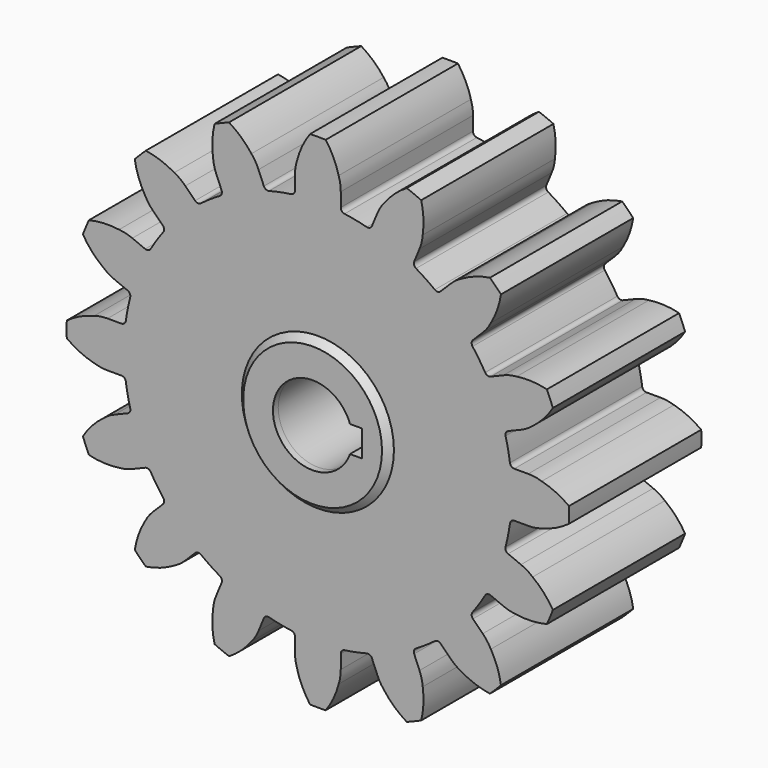
from build123d import *

# Parameters (mm, degrees)
F1_DEPTH = 25
F2_R     = 23
F3_DEPTH = 2
F4_SIZE  = 1.99999


# Not quite as in the source:
# - a fillet or chamfer is up to 0.001 mm smaller than in the source, because OpenCascade refuses the exact size
# - a pattern or mirror of a feature is missing from the dataset's text; its kind, count and spacing are read off the source's solid


with BuildPart() as f1:
    # F0 (on Front) → F1 (new body, symmetric)
    with BuildSketch(Plane.XZ):
        with BuildLine():
            ThreePointArc((-43.4371387857, 52.3183999575), (-47.5930049545, 54.262886018), (-52.0415397972, 55.3866241573))
            ThreePointArc((-52.0415397972, 55.3866241573), (-53.7401153702, 53.7401153702), (-55.3866241573, 52.0415397972))
            ThreePointArc((-55.3866241573, 52.0415397972), (-54.262886018, 47.5930049545), (-52.3183999575, 43.4371387857))
            ThreePointArc((-52.3183999575, 43.4371387857), (-51.237231337, 41.6673521086), (-49.8812173358, 40.0981814687))
            Line((-49.8812173358, 40.0981814687), (-46.908040594, 37.1250047269))
            ThreePointArc((-46.908040594, 37.1250047269), (-46.5216537829, 36.2761972334), (-46.7876742236, 35.3823280854))
            ThreePointArc((-46.7876742236, 35.3823280854), (-48.7740074577, 32.5897498689), (-50.593876495, 29.6859438322))
            ThreePointArc((-50.593876495, 29.6859438322), (-51.3179022902, 29.0981040781), (-52.2499619915, 29.1302543795))
            Line((-52.2499619915, 29.1302543795), (-56.1346046105, 30.7393260373))
            ThreePointArc((-56.1346046105, 30.7393260373), (-58.10325334, 31.3916240124), (-60.1520683466, 31.7132255318))
            ThreePointArc((-60.1520683466, 31.7132255318), (-64.7357106396, 31.9193152744), (-69.2756568986, 31.2551333587))
            ThreePointArc((-69.2756568986, 31.2551333587), (-70.2148444709, 29.0839408597), (-71.086003509, 26.8845700193))
            ThreePointArc((-71.086003509, 26.8845700193), (-68.3454242596, 23.2046956968), (-64.9585722571, 20.1092986034))
            ThreePointArc((-64.9585722571, 20.1092986034), (-63.2824346573, 18.8879742341), (-61.4291454693, 17.9571736892))
            Line((-61.4291454693, 17.9571736892), (-57.5445028504, 16.3481020315))
            ThreePointArc((-57.5445028504, 16.3481020315), (-56.862703419, 15.7117699924), (-56.7664053458, 14.7841409664))
            ThreePointArc((-56.7664053458, 14.7841409664), (-57.5328645485, 11.4439982895), (-58.1029658428, 8.0647975961))
            ThreePointArc((-58.1029658428, 8.0647975961), (-58.5469219213, 7.2446318025), (-59.4203361901, 6.9176510022))
            Line((-59.4203361901, 6.9176510022), (-63.6250430618, 6.9176510022))
            ThreePointArc((-63.6250430618, 6.9176510022), (-65.6934609577, 6.7669264976), (-67.7093907815, 6.28))
            ThreePointArc((-67.7093907815, 6.28), (-72.0229912104, 4.7163181297), (-75.9631832226, 2.3653318347))
            ThreePointArc((-75.9631832226, 2.3653318347), (-76, 0), (-75.9631832226, -2.3653318347))
            ThreePointArc((-75.9631832226, -2.3653318347), (-72.0229912104, -4.7163181297), (-67.7093907815, -6.28))
            ThreePointArc((-67.7093907815, -6.28), (-65.6934609577, -6.7669264976), (-63.6250430618, -6.9176510022))
            Line((-63.6250430618, -6.9176510022), (-59.4203361901, -6.9176510022))
            ThreePointArc((-59.4203361901, -6.9176510022), (-58.5469219213, -7.2446318025), (-58.1029658428, -8.0647975961))
            ThreePointArc((-58.1029658428, -8.0647975961), (-57.5328645485, -11.4439982895), (-56.7664053458, -14.7841409664))
            ThreePointArc((-56.7664053458, -14.7841409664), (-56.862703419, -15.7117699924), (-57.5445028504, -16.3481020315))
            Line((-57.5445028504, -16.3481020315), (-61.4291454693, -17.9571736892))
            ThreePointArc((-61.4291454693, -17.9571736892), (-63.2824346573, -18.8879742341), (-64.9585722571, -20.1092986034))
            ThreePointArc((-64.9585722571, -20.1092986034), (-68.3454242596, -23.2046956968), (-71.086003509, -26.8845700193))
            ThreePointArc((-71.086003509, -26.8845700193), (-70.2148444709, -29.0839408597), (-69.2756568986, -31.2551333587))
            ThreePointArc((-69.2756568986, -31.2551333587), (-64.7357106396, -31.9193152744), (-60.1520683466, -31.7132255318))
            ThreePointArc((-60.1520683466, -31.7132255318), (-58.10325334, -31.3916240124), (-56.1346046105, -30.7393260373))
            Line((-56.1346046105, -30.7393260373), (-52.2499619915, -29.1302543795))
            ThreePointArc((-52.2499619915, -29.1302543795), (-51.3179022902, -29.0981040781), (-50.593876495, -29.6859438322))
            ThreePointArc((-50.593876495, -29.6859438322), (-48.7740074577, -32.5897498689), (-46.7876742236, -35.3823280854))
            ThreePointArc((-46.7876742236, -35.3823280854), (-46.5216537829, -36.2761972334), (-46.908040594, -37.1250047269))
            Line((-46.908040594, -37.1250047269), (-49.8812173358, -40.0981814687))
            ThreePointArc((-49.8812173358, -40.0981814687), (-51.237231337, -41.6673521086), (-52.3183999575, -43.4371387857))
            ThreePointArc((-52.3183999575, -43.4371387857), (-54.262886018, -47.5930049545), (-55.3866241573, -52.0415397972))
            ThreePointArc((-55.3866241573, -52.0415397972), (-53.7401153702, -53.7401153702), (-52.0415397972, -55.3866241573))
            ThreePointArc((-52.0415397972, -55.3866241573), (-47.5930049545, -54.262886018), (-43.4371387857, -52.3183999575))
            ThreePointArc((-43.4371387857, -52.3183999575), (-41.6673521086, -51.237231337), (-40.0981814687, -49.8812173358))
            Line((-40.0981814687, -49.8812173358), (-37.1250047269, -46.908040594))
            ThreePointArc((-37.1250047269, -46.908040594), (-36.2761972334, -46.5216537829), (-35.3823280854, -46.7876742236))
            ThreePointArc((-35.3823280854, -46.7876742236), (-32.5897498689, -48.7740074577), (-29.6859438322, -50.593876495))
            ThreePointArc((-29.6859438322, -50.593876495), (-29.0981040781, -51.3179022902), (-29.1302543795, -52.2499619915))
            Line((-29.1302543795, -52.2499619915), (-30.7393260373, -56.1346046105))
            ThreePointArc((-30.7393260373, -56.1346046105), (-31.3916240124, -58.10325334), (-31.7132255318, -60.1520683466))
            ThreePointArc((-31.7132255318, -60.1520683466), (-31.9193152744, -64.7357106396), (-31.2551333587, -69.2756568986))
            ThreePointArc((-31.2551333587, -69.2756568986), (-29.0839408597, -70.2148444709), (-26.8845700193, -71.086003509))
            ThreePointArc((-26.8845700193, -71.086003509), (-23.2046956968, -68.3454242596), (-20.1092986034, -64.9585722571))
            ThreePointArc((-20.1092986034, -64.9585722571), (-18.8879742341, -63.2824346573), (-17.9571736892, -61.4291454693))
            Line((-17.9571736892, -61.4291454693), (-16.3481020315, -57.5445028504))
            ThreePointArc((-16.3481020315, -57.5445028504), (-15.7117699924, -56.862703419), (-14.7841409664, -56.7664053458))
            ThreePointArc((-14.7841409664, -56.7664053458), (-11.4439982895, -57.5328645485), (-8.0647975961, -58.1029658428))
            ThreePointArc((-8.0647975961, -58.1029658428), (-7.2446318025, -58.5469219213), (-6.9176510022, -59.4203361901))
            Line((-6.9176510022, -59.4203361901), (-6.9176510022, -63.6250430618))
            ThreePointArc((-6.9176510022, -63.6250430618), (-6.7669264976, -65.6934609577), (-6.28, -67.7093907815))
            ThreePointArc((-6.28, -67.7093907815), (-4.7163181297, -72.0229912104), (-2.3653318347, -75.9631832226))
            ThreePointArc((-2.3653318347, -75.9631832226), (0, -76), (2.3653318347, -75.9631832226))
            ThreePointArc((2.3653318347, -75.9631832226), (4.7163181297, -72.0229912104), (6.28, -67.7093907815))
            ThreePointArc((6.28, -67.7093907815), (6.7669264976, -65.6934609577), (6.9176510022, -63.6250430618))
            Line((6.9176510022, -63.6250430618), (6.9176510022, -59.4203361901))
            ThreePointArc((6.9176510022, -59.4203361901), (7.2446318025, -58.5469219213), (8.0647975961, -58.1029658428))
            ThreePointArc((8.0647975961, -58.1029658428), (11.4439982895, -57.5328645485), (14.7841409664, -56.7664053458))
            ThreePointArc((14.7841409664, -56.7664053458), (15.7117699924, -56.862703419), (16.3481020315, -57.5445028504))
            Line((16.3481020315, -57.5445028504), (17.9571736892, -61.4291454693))
            ThreePointArc((17.9571736892, -61.4291454693), (18.8879742341, -63.2824346573), (20.1092986034, -64.9585722571))
            ThreePointArc((20.1092986034, -64.9585722571), (23.2046956968, -68.3454242596), (26.8845700193, -71.086003509))
            ThreePointArc((26.8845700193, -71.086003509), (29.0839408597, -70.2148444709), (31.2551333587, -69.2756568986))
            ThreePointArc((31.2551333587, -69.2756568986), (31.9193152744, -64.7357106396), (31.7132255318, -60.1520683466))
            ThreePointArc((31.7132255318, -60.1520683466), (31.3916240124, -58.10325334), (30.7393260373, -56.1346046105))
            Line((30.7393260373, -56.1346046105), (29.1302543795, -52.2499619915))
            ThreePointArc((29.1302543795, -52.2499619915), (29.0981040781, -51.3179022902), (29.6859438322, -50.593876495))
            ThreePointArc((29.6859438322, -50.593876495), (32.5897498689, -48.7740074577), (35.3823280854, -46.7876742236))
            ThreePointArc((35.3823280854, -46.7876742236), (36.2761972334, -46.5216537829), (37.1250047269, -46.908040594))
            Line((37.1250047269, -46.908040594), (40.0981814687, -49.8812173358))
            ThreePointArc((40.0981814687, -49.8812173358), (41.6673521086, -51.237231337), (43.4371387857, -52.3183999575))
            ThreePointArc((43.4371387857, -52.3183999575), (47.5930049545, -54.262886018), (52.0415397972, -55.3866241573))
            ThreePointArc((52.0415397972, -55.3866241573), (53.7401153702, -53.7401153702), (55.3866241573, -52.0415397972))
            ThreePointArc((55.3866241573, -52.0415397972), (54.262886018, -47.5930049545), (52.3183999575, -43.4371387857))
            ThreePointArc((52.3183999575, -43.4371387857), (51.237231337, -41.6673521086), (49.8812173358, -40.0981814687))
            Line((49.8812173358, -40.0981814687), (46.908040594, -37.1250047269))
            ThreePointArc((46.908040594, -37.1250047269), (46.5216537829, -36.2761972334), (46.7876742236, -35.3823280854))
            ThreePointArc((46.7876742236, -35.3823280854), (48.7740074577, -32.5897498689), (50.593876495, -29.6859438322))
            ThreePointArc((50.593876495, -29.6859438322), (51.3179022902, -29.0981040781), (52.2499619915, -29.1302543795))
            Line((52.2499619915, -29.1302543795), (56.1346046105, -30.7393260373))
            ThreePointArc((56.1346046105, -30.7393260373), (58.10325334, -31.3916240124), (60.1520683466, -31.7132255318))
            ThreePointArc((60.1520683466, -31.7132255318), (64.7357106396, -31.9193152744), (69.2756568986, -31.2551333587))
            ThreePointArc((69.2756568986, -31.2551333587), (70.2148444709, -29.0839408597), (71.086003509, -26.8845700193))
            ThreePointArc((71.086003509, -26.8845700193), (68.3454242596, -23.2046956968), (64.9585722571, -20.1092986034))
            ThreePointArc((64.9585722571, -20.1092986034), (63.2824346573, -18.8879742341), (61.4291454693, -17.9571736892))
            Line((61.4291454693, -17.9571736892), (57.5445028504, -16.3481020315))
            ThreePointArc((57.5445028504, -16.3481020315), (56.862703419, -15.7117699924), (56.7664053458, -14.7841409664))
            ThreePointArc((56.7664053458, -14.7841409664), (57.5328645485, -11.4439982895), (58.1029658428, -8.0647975961))
            ThreePointArc((58.1029658428, -8.0647975961), (58.5469219213, -7.2446318025), (59.4203361901, -6.9176510022))
            Line((59.4203361901, -6.9176510022), (63.6250430618, -6.9176510022))
            ThreePointArc((63.6250430618, -6.9176510022), (65.6934609577, -6.7669264976), (67.7093907815, -6.28))
            ThreePointArc((67.7093907815, -6.28), (72.0229912104, -4.7163181297), (75.9631832226, -2.3653318347))
            ThreePointArc((75.9631832226, -2.3653318347), (76, 0), (75.9631832226, 2.3653318347))
            ThreePointArc((75.9631832226, 2.3653318347), (72.0229912104, 4.7163181297), (67.7093907815, 6.28))
            ThreePointArc((67.7093907815, 6.28), (65.6934609577, 6.7669264976), (63.6250430618, 6.9176510022))
            Line((63.6250430618, 6.9176510022), (59.4203361901, 6.9176510022))
            ThreePointArc((59.4203361901, 6.9176510022), (58.5469219213, 7.2446318025), (58.1029658428, 8.0647975961))
            ThreePointArc((58.1029658428, 8.0647975961), (57.5328645485, 11.4439982895), (56.7664053458, 14.7841409664))
            ThreePointArc((56.7664053458, 14.7841409664), (56.862703419, 15.7117699924), (57.5445028504, 16.3481020315))
            Line((57.5445028504, 16.3481020315), (61.4291454693, 17.9571736892))
            ThreePointArc((61.4291454693, 17.9571736892), (63.2824346573, 18.8879742341), (64.9585722571, 20.1092986034))
            ThreePointArc((64.9585722571, 20.1092986034), (68.3454242596, 23.2046956968), (71.086003509, 26.8845700193))
            ThreePointArc((71.086003509, 26.8845700193), (70.2148444709, 29.0839408597), (69.2756568986, 31.2551333587))
            ThreePointArc((69.2756568986, 31.2551333587), (64.7357106396, 31.9193152744), (60.1520683466, 31.7132255318))
            ThreePointArc((60.1520683466, 31.7132255318), (58.10325334, 31.3916240124), (56.1346046105, 30.7393260373))
            Line((56.1346046105, 30.7393260373), (52.2499619915, 29.1302543795))
            ThreePointArc((52.2499619915, 29.1302543795), (51.3179022902, 29.0981040781), (50.593876495, 29.6859438322))
            ThreePointArc((50.593876495, 29.6859438322), (48.7740074577, 32.5897498689), (46.7876742236, 35.3823280854))
            ThreePointArc((46.7876742236, 35.3823280854), (46.5216537829, 36.2761972334), (46.908040594, 37.1250047269))
            Line((46.908040594, 37.1250047269), (49.8812173358, 40.0981814687))
            ThreePointArc((49.8812173358, 40.0981814687), (51.237231337, 41.6673521086), (52.3183999575, 43.4371387857))
            ThreePointArc((52.3183999575, 43.4371387857), (54.262886018, 47.5930049545), (55.3866241573, 52.0415397972))
            ThreePointArc((55.3866241573, 52.0415397972), (53.7401153702, 53.7401153702), (52.0415397972, 55.3866241573))
            ThreePointArc((52.0415397972, 55.3866241573), (47.5930049545, 54.262886018), (43.4371387857, 52.3183999575))
            ThreePointArc((43.4371387857, 52.3183999575), (41.6673521086, 51.237231337), (40.0981814687, 49.8812173358))
            Line((40.0981814687, 49.8812173358), (37.1250047269, 46.908040594))
            ThreePointArc((37.1250047269, 46.908040594), (36.2761972334, 46.5216537829), (35.3823280854, 46.7876742236))
            ThreePointArc((35.3823280854, 46.7876742236), (32.5897498689, 48.7740074577), (29.6859438322, 50.593876495))
            ThreePointArc((29.6859438322, 50.593876495), (29.0981040781, 51.3179022902), (29.1302543795, 52.2499619915))
            Line((29.1302543795, 52.2499619915), (30.7393260373, 56.1346046105))
            ThreePointArc((30.7393260373, 56.1346046105), (31.3916240124, 58.10325334), (31.7132255318, 60.1520683466))
            ThreePointArc((31.7132255318, 60.1520683466), (31.9193152744, 64.7357106396), (31.2551333587, 69.2756568986))
            ThreePointArc((31.2551333587, 69.2756568986), (29.0839408597, 70.2148444709), (26.8845700193, 71.086003509))
            ThreePointArc((26.8845700193, 71.086003509), (23.2046956968, 68.3454242596), (20.1092986034, 64.9585722571))
            ThreePointArc((20.1092986034, 64.9585722571), (18.8879742341, 63.2824346573), (17.9571736892, 61.4291454693))
            Line((17.9571736892, 61.4291454693), (16.3481020315, 57.5445028504))
            ThreePointArc((16.3481020315, 57.5445028504), (15.7117699924, 56.862703419), (14.7841409664, 56.7664053458))
            ThreePointArc((14.7841409664, 56.7664053458), (11.4439982895, 57.5328645485), (8.0647975961, 58.1029658428))
            ThreePointArc((8.0647975961, 58.1029658428), (7.2446318025, 58.5469219213), (6.9176510022, 59.4203361901))
            Line((6.9176510022, 59.4203361901), (6.9176510022, 63.6250430618))
            ThreePointArc((6.9176510022, 63.6250430618), (6.7669264976, 65.6934609577), (6.28, 67.7093907815))
            ThreePointArc((6.28, 67.7093907815), (4.7163181297, 72.0229912104), (2.3653318347, 75.9631832226))
            ThreePointArc((2.3653318347, 75.9631832226), (0, 76), (-2.3653318347, 75.9631832226))
            ThreePointArc((-2.3653318347, 75.9631832226), (-4.7163181297, 72.0229912104), (-6.28, 67.7093907815))
            ThreePointArc((-6.28, 67.7093907815), (-6.7669264976, 65.6934609577), (-6.9176510022, 63.6250430618))
            Line((-6.9176510022, 63.6250430618), (-6.9176510022, 59.4203361901))
            ThreePointArc((-6.9176510022, 59.4203361901), (-7.2446318025, 58.5469219213), (-8.0647975961, 58.1029658428))
            ThreePointArc((-8.0647975961, 58.1029658428), (-11.4439982895, 57.5328645485), (-14.7841409664, 56.7664053458))
            ThreePointArc((-14.7841409664, 56.7664053458), (-15.7117699924, 56.862703419), (-16.3481020315, 57.5445028504))
            Line((-16.3481020315, 57.5445028504), (-17.9571736892, 61.4291454693))
            ThreePointArc((-17.9571736892, 61.4291454693), (-18.8879742341, 63.2824346573), (-20.1092986034, 64.9585722571))
            ThreePointArc((-20.1092986034, 64.9585722571), (-23.2046956968, 68.3454242596), (-26.8845700193, 71.086003509))
            ThreePointArc((-26.8845700193, 71.086003509), (-29.0839408597, 70.2148444709), (-31.2551333587, 69.2756568986))
            ThreePointArc((-31.2551333587, 69.2756568986), (-31.9193152744, 64.7357106396), (-31.7132255318, 60.1520683466))
            ThreePointArc((-31.7132255318, 60.1520683466), (-31.3916240124, 58.10325334), (-30.7393260373, 56.1346046105))
            Line((-30.7393260373, 56.1346046105), (-29.1302543795, 52.2499619915))
            ThreePointArc((-29.1302543795, 52.2499619915), (-29.0981040781, 51.3179022902), (-29.6859438322, 50.593876495))
            ThreePointArc((-29.6859438322, 50.593876495), (-32.5897498689, 48.7740074577), (-35.3823280854, 46.7876742236))
            ThreePointArc((-35.3823280854, 46.7876742236), (-36.2761972334, 46.5216537829), (-37.1250047269, 46.908040594))
            Line((-37.1250047269, 46.908040594), (-40.0981814687, 49.8812173358))
            ThreePointArc((-40.0981814687, 49.8812173358), (-41.6673521086, 51.237231337), (-43.4371387857, 52.3183999575))
        make_face()
        with BuildLine():
            ThreePointArc((-12, 0), (-2.0292237447, 11.8271827158), (11.313708499, 4))
            Line((11.313708499, 4), (15, 4))
            Line((15, 4), (15, 0))
            Line((15, 0), (15, -4))
            Line((15, -4), (11.313708499, -4))
            ThreePointArc((11.313708499, -4), (-2.0292237447, -11.8271827158), (-12, 0))
        make_face(mode=Mode.SUBTRACT)
    extrude(amount=F1_DEPTH, both=True)

    # F2 (on face) → F3 (join)
    with BuildSketch(Plane.XZ.offset(25)):
        Circle(F2_R)
        with BuildLine():
            ThreePointArc((11.313708499, -4), (-12, 0), (11.313708499, 4))
            Line((11.313708499, 4), (15, 4))
            Line((15, 4), (15, -4))
            Line((15, -4), (11.313708499, -4))
        make_face(mode=Mode.SUBTRACT)
    f3 = extrude(amount=F3_DEPTH)

    # F3_copies: F3 across plane
    add(f3.mirror(Plane.ZX))

    # F4 (size 2 in the source; OpenCascade refuses exactly that, so slightly less here)
    f4_edges = [f1.edges().sort_by_distance(p)[0] for p in [
        (-23, -27, 0),
        (-23, 27, 0),
    ]]
    chamfer(f4_edges, length=F4_SIZE)


solid = f1.part
